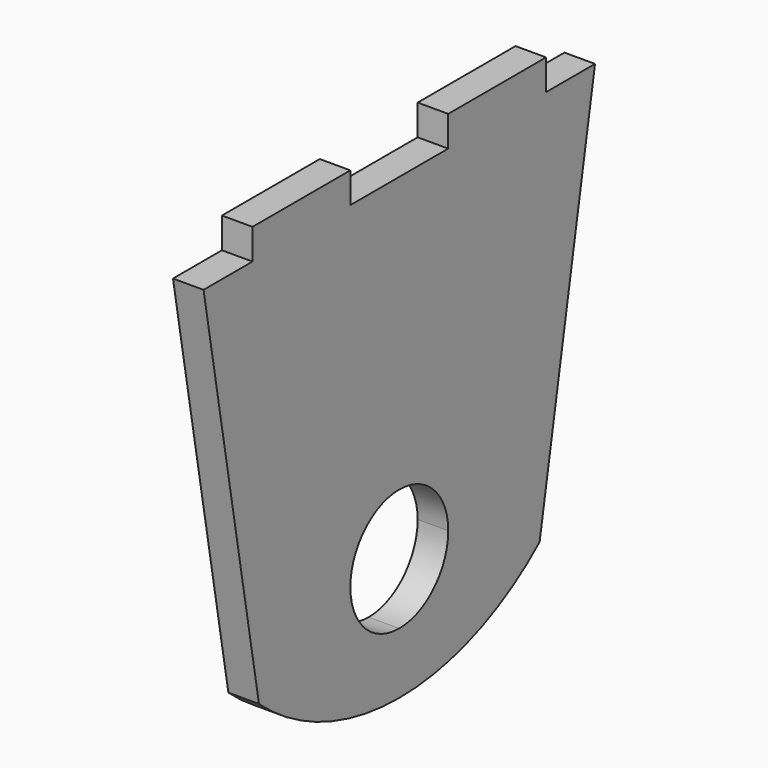
from build123d import *

# Parameters (mm, degrees)
F1_DEPTH = 6.35
F2_W     = 12.7
F2_H     = 6.35
F3_DEPTH = 25.4
F5_DEPTH = 6.351


# Not quite as in the source:
# - a feature names something its author has since deleted; it is built from what else it names


with BuildPart() as f1:
    # F0 (on Right) → F1 (new body)
    with BuildSketch(Plane.YZ):
        with BuildLine():
            Line((50.8, 0), (0, 0))
            Line((0, 0), (0, -6.35))
            Line((0, -6.35), (14.3783799252, -87.8938446653))
            ThreePointArc((14.3783799252, -87.8938446653), (31.3423979963, -98.0600456848), (50.8, -101.6))
            Line((50.8, -101.6), (50.8, 0))
        make_face()
        with BuildLine():
            Line((101.6, 0), (50.8, 0))
            Line((50.8, 0), (50.8, -101.6))
            ThreePointArc((50.8, -101.6), (70.2576020037, -98.0600456848), (87.2216200748, -87.8938446653))
            Line((87.2216200748, -87.8938446653), (101.6, -6.35))
            Line((101.6, -6.35), (101.6, 0))
        make_face()
    extrude(amount=F1_DEPTH)

    # F2 (on face) → F3 (cut)
    with BuildSketch(Plane.YZ.offset(6.35)):
        with Locations((95.25, -3.175)):
            Rectangle(F2_W, F2_H)
        with Locations((44.45, -3.175)):
            Rectangle(F2_W, F2_H)
        with Locations((6.35, -3.175)):
            Rectangle(F2_W, F2_H)
        with Locations((57.15, -3.175)):
            Rectangle(F2_W, F2_H)
    extrude(amount=-F3_DEPTH, mode=Mode.SUBTRACT)

    # F4 (on face) → F5 (cut, through all)
    with BuildSketch(Plane.YZ.offset(6.35)):
        with BuildLine():
            Line((50.8, -88.9), (50.8, -76.2))
            Line((50.8, -76.2), (38.1, -76.2))
            ThreePointArc((38.1, -76.2), (41.8197438789, -85.1802561211), (50.8, -88.9))
        make_face()
        with BuildLine():
            Line((50.8, -76.2), (63.5, -76.2))
            ThreePointArc((63.5, -76.2), (59.7802561211, -67.2197438789), (50.8, -63.5))
            Line((50.8, -63.5), (50.8, -76.2))
        make_face()
        with BuildLine():
            ThreePointArc((50.8, -88.9), (59.7802561211, -85.1802561211), (63.5, -76.2))
            Line((63.5, -76.2), (50.8, -76.2))
            Line((50.8, -76.2), (50.8, -88.9))
        make_face()
        with BuildLine():
            Line((38.1, -76.2), (50.8, -76.2))
            Line((50.8, -76.2), (50.8, -63.5))
            ThreePointArc((50.8, -63.5), (41.8197438789, -67.2197438789), (38.1, -76.2))
        make_face()
    extrude(amount=-F5_DEPTH, mode=Mode.SUBTRACT)


solid = f1.part
